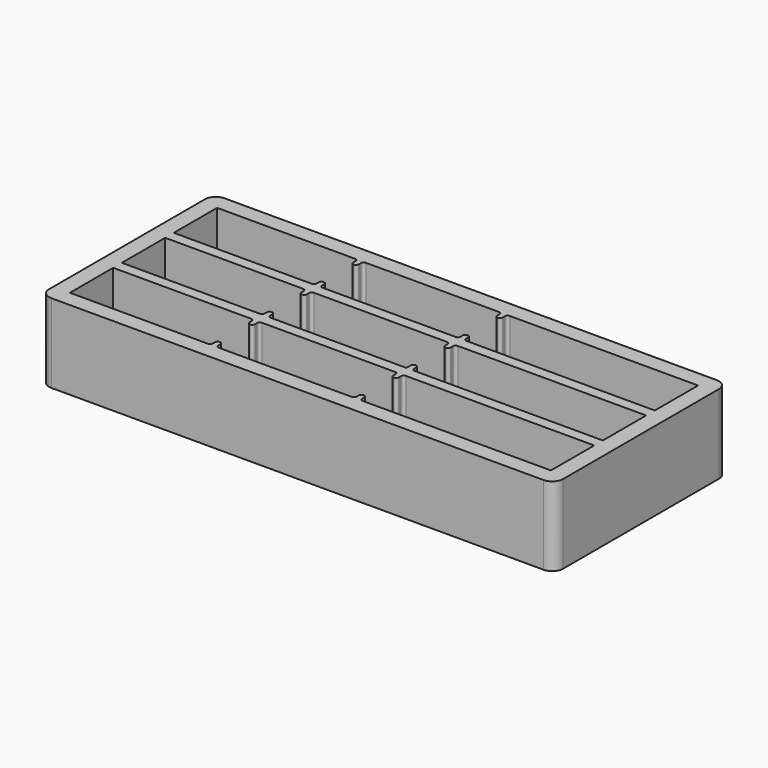
from build123d import *

# Parameters (mm, degrees)
F0_W     = 95
F0_H     = 40
F1_DEPTH = 14.6
F2_W     = 88.9
F2_H     = 10
F3_DEPTH = 12.6
F4_W     = 1
F4_H     = 1.5
F5_DEPTH = 12.6
F6_R     = 3.5
F7_DEPTH = 14.601
F8_R     = 2
F9_R     = 0.49999


# Not quite as in the source:
# - a fillet or chamfer is up to 0.001 mm smaller than in the source, because OpenCascade refuses the exact size


with BuildPart() as f1:
    # F0 (on Top) → F1 (new body)
    with BuildSketch(Plane.XY):
        Rectangle(F0_W, F0_H)
    extrude(amount=F1_DEPTH)

    # F2 (on face) → F3 (cut)
    with BuildSketch(Plane.XY.offset(14.6)):
        with Locations((0, 12)):
            Rectangle(F2_W, F2_H)
        Rectangle(F2_W, F2_H)
        with Locations((0, -12)):
            Rectangle(F2_W, F2_H)
    extrude(amount=-F3_DEPTH, mode=Mode.SUBTRACT)

    # F4 (on face) → F5 (join, through all)
    with BuildSketch(Plane.XY.offset(14.6)):
        with Locations((-17.95, 16.25)):
            Rectangle(F4_W, F4_H)
        with Locations((8.65, 16.25)):
            Rectangle(F4_W, F4_H)
        with Locations((8.65, 7.75)):
            Rectangle(F4_W, F4_H)
        with Locations((-17.95, 7.75)):
            Rectangle(F4_W, F4_H)
        with Locations((-17.95, 4.25)):
            Rectangle(F4_W, F4_H)
        with Locations((8.65, 4.25)):
            Rectangle(F4_W, F4_H)
        with Locations((8.65, -16.25)):
            Rectangle(F4_W, F4_H)
        with Locations((-17.95, -16.25)):
            Rectangle(F4_W, F4_H)
        with Locations((-17.95, -4.25)):
            Rectangle(F4_W, F4_H)
        with Locations((-17.95, -7.75)):
            Rectangle(F4_W, F4_H)
        with Locations((8.65, -4.25)):
            Rectangle(F4_W, F4_H)
        with Locations((8.65, -7.75)):
            Rectangle(F4_W, F4_H)
    extrude(amount=-F5_DEPTH)

    # F6 (on face) → F7 (cut, through all)
    with BuildSketch(Plane.XY.offset(14.6)):
        with Locations((-39.55, 12)):
            Circle(F6_R)
        with Locations((-31.45, 12)):
            Circle(F6_R)
        with Locations((-23.35, 12)):
            Circle(F6_R)
        with Locations((-12.55, 12)):
            Circle(F6_R)
        with Locations((-4.45, 12)):
            Circle(F6_R)
        with Locations((3.65, 12)):
            Circle(F6_R)
        with Locations((14.65, 12)):
            Circle(F6_R)
        with Locations((22.75, 12)):
            Circle(F6_R)
        with Locations((30.85, 12)):
            Circle(F6_R)
        with Locations((38.95, 12)):
            Circle(F6_R)
        with Locations((-39.55, 0)):
            Circle(F6_R)
        with Locations((-31.45, 0)):
            Circle(F6_R)
        with Locations((-23.35, 0)):
            Circle(F6_R)
        with Locations((-12.55, 0)):
            Circle(F6_R)
        with Locations((-4.45, 0)):
            Circle(F6_R)
        with Locations((3.65, 0)):
            Circle(F6_R)
        with Locations((14.65, 0)):
            Circle(F6_R)
        with Locations((22.75, 0)):
            Circle(F6_R)
        with Locations((30.85, 0)):
            Circle(F6_R)
        with Locations((38.95, 0)):
            Circle(F6_R)
        with Locations((-39.55, -12)):
            Circle(F6_R)
        with Locations((-31.45, -12)):
            Circle(F6_R)
        with Locations((-23.35, -12)):
            Circle(F6_R)
        with Locations((-12.55, -12)):
            Circle(F6_R)
        with Locations((-4.45, -12)):
            Circle(F6_R)
        with Locations((3.65, -12)):
            Circle(F6_R)
        with Locations((14.65, -12)):
            Circle(F6_R)
        with Locations((22.75, -12)):
            Circle(F6_R)
        with Locations((30.85, -12)):
            Circle(F6_R)
        with Locations((38.95, -12)):
            Circle(F6_R)
    extrude(amount=-F7_DEPTH, mode=Mode.SUBTRACT)

    # F8
    f8_edges = [f1.edges().sort_by_distance(p)[0] for p in [
        (-47.5, -20, 7.3),
        (47.5, -20, 7.3),
        (47.5, 20, 7.3),
        (-47.5, 20, 7.3),
    ]]
    fillet(f8_edges, radius=F8_R)

    # F9 (radius 0.5 in the source; OpenCascade refuses exactly that, so slightly less here)
    f9_edges = [f1.edges().sort_by_distance(p)[0] for p in [
        (-18.45, 17, 8.3),
        (-18.45, 15.5, 8.3),
        (-17.45, 15.5, 8.3),
        (8.15, 17, 8.3),
        (8.15, 15.5, 8.3),
        (9.15, 15.5, 8.3),
        (8.15, 8.5, 8.3),
        (-18.45, 8.5, 8.3),
        (-18.45, 5, 8.3),
        (-18.45, 3.5, 8.3),
        (-17.45, 3.5, 8.3),
        (8.15, 5, 8.3),
        (8.15, 3.5, 8.3),
        (-18.45, -3.5, 8.3),
        (8.15, -3.5, 8.3),
        (-18.45, -8.5, 8.3),
        (-17.45, -8.5, 8.3),
        (-18.45, -7, 8.3),
        (8.15, -7, 8.3),
        (8.15, -8.5, 8.3),
        (9.15, -8.5, 8.3),
        (8.15, -15.5, 8.3),
        (-18.45, -15.5, 8.3),
        (-17.45, -17, 8.3),
        (-17.45, -15.5, 8.3),
        (9.15, -17, 8.3),
        (9.15, -15.5, 8.3),
        (9.15, -5, 8.3),
        (9.15, -3.5, 8.3),
        (9.15, 8.5, 8.3),
        (9.15, 3.5, 8.3),
        (-17.45, -3.5, 8.3),
        (-17.45, -5, 8.3),
        (-17.45, 8.5, 8.3),
        (-17.45, 7, 8.3),
        (9.15, 7, 8.3),
        (8.15, -17, 8.3),
        (-18.45, -17, 8.3),
        (-18.45, -5, 8.3),
        (-18.45, 7, 8.3),
        (8.15, 7, 8.3),
        (9.15, -7, 8.3),
        (9.15, 5, 8.3),
        (-17.45, 5, 8.3),
        (-17.45, -7, 8.3),
        (9.15, 17, 8.3),
        (-17.45, 17, 8.3),
    ]]
    fillet(f9_edges, radius=F9_R)


solid = f1.part
